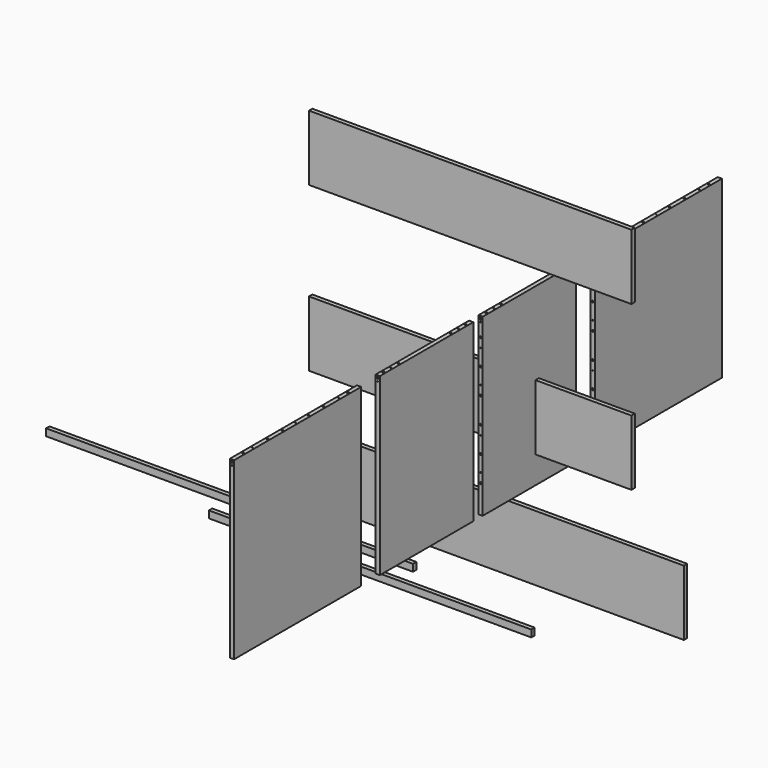
from build123d import *

# Parameters (mm, degrees)
F0_W      = 500
F0_H      = 750
F3_DEPTH  = 18
F4_D      = 4.5
F4_DEPTH  = 10
F4_TIP    = 1.3519363928
F5_D      = 8
F5_DEPTH  = 10
F5_TIP    = 2.4034424761
F6_D      = 5
F6_DEPTH  = 10
F6_TIP    = 1.5021515476
F7_W      = 680
F7_H      = 750
F8_DEPTH  = 18
F10_D     = 4
F11_D     = 8
F12_W     = 1570
F12_H     = 280
F13_DEPTH = 18
F14_W     = 1570
F14_H     = 280
F15_DEPTH = 18
F14_W_2   = 1380
F18_D     = 8
F18_DEPTH = 20
F18_TIP   = 2.4034424761
F19_D     = 5
F19_DEPTH = 60
F19_TIP   = 1.5021515476
F21_D     = 4
F21_DEPTH = 40
F21_TIP   = 1.2017212381
F22_D     = 8
F22_DEPTH = 30
F22_TIP   = 2.4034424761
F24_W     = 1570
F24_H     = 30
F25_DEPTH = 18
F27_D     = 8
F27_DEPTH = 10
F27_TIP   = 2.4034424761
F28_D     = 4
F28_DEPTH = 10
F28_TIP   = 1.2017212381
F29_W     = 1380
F29_H     = 30
F30_DEPTH = 18
F32_D     = 4
F32_DEPTH = 10
F32_TIP   = 1.2017212381
F33_D     = 8
F33_DEPTH = 10
F33_TIP   = 2.4034424761
F35_D     = 8
F35_DEPTH = 20
F35_TIP   = 2.4034424761
F36_D     = 4
F36_DEPTH = 40
F36_TIP   = 1.2017212381
F38_D     = 8
F39_D     = 4
F41_D     = 4
F41_DEPTH = 40
F41_START = 600
F41_TIP   = 1.2017212381
F42_D     = 8
F42_DEPTH = 25
F42_START = 600
F42_TIP   = 2.4034424761
F45_D     = 8
F45_DEPTH = 10
F45_TIP   = 2.4034424761
F46_D     = 8
F46_DEPTH = 10
F46_TIP   = 2.4034424761
F47_D     = 4
F47_DEPTH = 12
F47_TIP   = 1.2017212381
F48_D     = 4
F48_DEPTH = 12
F48_TIP   = 1.2017212381


# Not quite as in the source:
# - a feature names something its author has since deleted; it is built from what else it names


with BuildPart() as f3:
    # F0 (on Right) → F3 (new body)
    with BuildSketch(Plane.YZ):
        with Locations((-50.6659869477, 62.4944338164)):
            Rectangle(F0_W, F0_H)
    extrude(amount=F3_DEPTH)

    # F4
    with Locations(Plane(origin=(0, 0, 0), x_dir=(0, 1, 0), z_dir=(-1, 0, 0))):
        with Locations((114.6340130523, 182.5055661836), (50.6340130523, 182.5055661836), (-162.4159869477, 182.5055661836), (-226.4159869477, 182.5055661836), (114.6340130523, 12.5055661836), (50.6340130523, 12.5055661836), (-162.4159869477, 12.5055661836), (-226.4159869477, 12.5055661836), (-226.4159869477, -157.4944338164), (-162.4159869477, -157.4944338164), (114.6340130523, -157.4944338164), (50.6340130523, -157.4944338164)):
            Hole(F4_D / 2, depth=F4_DEPTH)
            with Locations((0, 0, -(F4_DEPTH + F4_TIP / 2))):  # 118° drill point
                Cone(0, F4_D / 2, F4_TIP, mode=Mode.SUBTRACT)

    # F5
    with Locations(Plane(origin=(0, 0, 0), x_dir=(0, 1, 0), z_dir=(-1, 0, 0))):
        with Locations((-250.6659869477, 257.5055661836), (-150.6659869477, 257.5055661836), (-50.6659869477, 257.5055661836), (49.3340130523, 257.5055661836), (149.3340130523, 257.5055661836), (149.3340130523, -232.4944338164), (49.3340130523, -232.4944338164), (-50.6659869477, -232.4944338164), (-250.6659869477, -232.4944338164), (-150.6659869477, -232.4944338164)):
            Hole(F5_D / 2, depth=F5_DEPTH)
            with Locations((0, 0, -(F5_DEPTH + F5_TIP / 2))):  # 118° drill point
                Cone(0, F5_D / 2, F5_TIP, mode=Mode.SUBTRACT)

    # F6
    with Locations(Plane(origin=(0, 0, 0), x_dir=(0, 1, 0), z_dir=(-1, 0, 0))):
        with Locations((99.3340130523, 257.5055661836), (-200.6659869477, 257.5055661836), (99.3340130523, -232.4944338164), (-200.6659869477, -232.4944338164)):
            Hole(F6_D / 2, depth=F6_DEPTH)
            with Locations((0, 0, -(F6_DEPTH + F6_TIP / 2))):  # 118° drill point
                Cone(0, F6_D / 2, F6_TIP, mode=Mode.SUBTRACT)

    # F18
    with Locations(Plane.XY.offset(437.4944338164)):
        with Locations((9, 169.3340130523), (9, 89.3340130523), (9, -190.6659869477), (9, -270.6659869477)):
            Hole(F18_D / 2, depth=F18_DEPTH)
            with Locations((0, 0, -(F18_DEPTH + F18_TIP / 2))):  # 118° drill point
                Cone(0, F18_D / 2, F18_TIP, mode=Mode.SUBTRACT)

    # F19
    with Locations(Plane.XY.offset(437.4944338164)):
        with Locations((9, 129.3340130523), (9, -230.6659869477)):
            Hole(F19_D / 2, depth=F19_DEPTH)
            with Locations((0, 0, -(F19_DEPTH + F19_TIP / 2))):  # 118° drill point
                Cone(0, F19_D / 2, F19_TIP, mode=Mode.SUBTRACT)

    # F35
    with Locations(Plane.XZ.offset(300.6659869477)):
        with Locations((9, 357.4944338164), (9, 247.4944338164), (9, 137.4944338164), (9, -192.5055661836), (9, -82.5055661836), (9, 27.4944338164)):
            Hole(F35_D / 2, depth=F35_DEPTH)
            with Locations((0, 0, -(F35_DEPTH + F35_TIP / 2))):  # 118° drill point
                Cone(0, F35_D / 2, F35_TIP, mode=Mode.SUBTRACT)

    # F36
    with Locations(Plane.XZ.offset(300.6659869477)):
        with Locations((9, 317.4944338164), (9, 177.4944338164), (9, -12.5055661836), (9, -152.5055661836)):
            Hole(F36_D / 2, depth=F36_DEPTH)
            with Locations((0, 0, -(F36_DEPTH + F36_TIP / 2))):  # 118° drill point
                Cone(0, F36_D / 2, F36_TIP, mode=Mode.SUBTRACT)

    # F38 (through all)
    with Locations(Plane(origin=(0, 199.3340130523, 0), x_dir=(-1, 0, 0), z_dir=(0, 1, 0))):
        with Locations((-9, 428.4944338164)):
            Hole(F38_D / 2)

    # F39 (through all)
    with Locations(Plane(origin=(0, 199.3340130523, 0), x_dir=(-1, 0, 0), z_dir=(0, 1, 0))):
        with Locations((-9, 414.9944338164)):
            Hole(F39_D / 2)


with BuildPart() as f8:
    # F7 (on Right) → F8 (new body)
    with BuildSketch(Plane.YZ):
        with Locations((639.3340130523, 62.4944338164)):
            Rectangle(F7_W, F7_H)
    extrude(amount=F8_DEPTH)

    # F10 (through all)
    with Locations(Plane(origin=(0, 979.3340130523, 0), x_dir=(-1, 0, 0), z_dir=(0, 1, 0))):
        with Locations((-9, 414.9944338164)):
            Hole(F10_D / 2)

    # F11 (through all)
    with Locations(Plane(origin=(0, 979.3340130523, 0), x_dir=(-1, 0, 0), z_dir=(0, 1, 0))):
        with Locations((-9, 428.4944338164)):
            Hole(F11_D / 2)

    # F21
    with Locations(Plane.XY.offset(437.4944338164)):
        with Locations((9, 869.3340130523), (9, 639.3340130523), (9, 409.3340130523)):
            Hole(F21_D / 2, depth=F21_DEPTH)
            with Locations((0, 0, -(F21_DEPTH + F21_TIP / 2))):  # 118° drill point
                Cone(0, F21_D / 2, F21_TIP, mode=Mode.SUBTRACT)

    # F22
    with Locations(Plane.XY.offset(437.4944338164)):
        with Locations((9, 359.3340130523), (9, 489.3340130523), (9, 569.3340130523), (9, 709.3340130523), (9, 789.3340130523), (9, 919.3340130523)):
            Hole(F22_D / 2, depth=F22_DEPTH)
            with Locations((0, 0, -(F22_DEPTH + F22_TIP / 2))):  # 118° drill point
                Cone(0, F22_D / 2, F22_TIP, mode=Mode.SUBTRACT)

    # F41
    # its depths count from where the whole tool has entered the part; down to there all is cleared
    with Locations(Plane.XZ.offset(300.6659869477)):
        with Locations((9, 317.4944338164), (9, 177.4944338164), (9, -12.5055661836), (9, -152.5055661836)):
            Hole(F41_D / 2, depth=F41_START)
    with Locations(Plane.XZ.offset(300.6659869477).offset(-F41_START)):
        with Locations((9, 317.4944338164), (9, 177.4944338164), (9, -12.5055661836), (9, -152.5055661836)):
            Hole(F41_D / 2, depth=F41_DEPTH)
            with Locations((0, 0, -(F41_DEPTH + F41_TIP / 2))):  # 118° drill point
                Cone(0, F41_D / 2, F41_TIP, mode=Mode.SUBTRACT)

    # F42
    # its depths count from where the whole tool has entered the part; down to there all is cleared
    with Locations(Plane.XZ.offset(300.6659869477)):
        with Locations((9, 357.4944338164), (9, 247.4944338164), (9, 137.4944338164), (9, 27.4944338164), (9, -82.5055661836), (9, -192.5055661836)):
            Hole(F42_D / 2, depth=F42_START)
    with Locations(Plane.XZ.offset(300.6659869477).offset(-F42_START)):
        with Locations((9, 357.4944338164), (9, 247.4944338164), (9, 137.4944338164), (9, 27.4944338164), (9, -82.5055661836), (9, -192.5055661836)):
            Hole(F42_D / 2, depth=F42_DEPTH)
            with Locations((0, 0, -(F42_DEPTH + F42_TIP / 2))):  # 118° drill point
                Cone(0, F42_D / 2, F42_TIP, mode=Mode.SUBTRACT)


with BuildPart() as f13:
    # F12 (on Front) → F13 (new body)
    with BuildSketch(Plane.XZ):
        with Locations((-131.9031941891, -548.7108457167)):
            Rectangle(F12_W, F12_H)
    extrude(amount=F13_DEPTH)

    # F46
    with Locations(Plane(origin=(0, 0, 0), x_dir=(-1, 0, 0), z_dir=(0, 1, 0))):
        with Locations((-644.0968058109, -438.7108457167), (-644.0968058109, -548.7108457167), (-644.0968058109, -658.7108457167), (907.9031941891, -438.7108457167), (907.9031941891, -548.7108457167), (907.9031941891, -658.7108457167)):
            Hole(F46_D / 2, depth=F46_DEPTH)
            with Locations((0, 0, -(F46_DEPTH + F46_TIP / 2))):  # 118° drill point
                Cone(0, F46_D / 2, F46_TIP, mode=Mode.SUBTRACT)

    # F47
    with Locations(Plane(origin=(0, 0, 0), x_dir=(-1, 0, 0), z_dir=(0, 1, 0))):
        with Locations((-644.0968058109, -478.7108457167), (-644.0968058109, -618.7108457167), (907.9031941891, -618.7108457167), (907.9031941891, -478.7108457167)):
            Hole(F47_D / 2, depth=F47_DEPTH)
            with Locations((0, 0, -(F47_DEPTH + F47_TIP / 2))):  # 118° drill point
                Cone(0, F47_D / 2, F47_TIP, mode=Mode.SUBTRACT)


with BuildPart() as f15:
    # F14 (on Front) → F15 (new body)
    with BuildSketch(Plane.XZ):
        with Locations((-131.9031941891, -548.7108457167)):
            Rectangle(F14_W, F14_H)
    extrude(amount=F15_DEPTH)


with BuildPart() as f15b:
    # F14 (on Front) → F15, piece 2 (new body)
    with BuildSketch(Plane.XZ):
        with Locations((-261.5306949615, -56.0900127888)):
            Rectangle(F14_W_2, F14_H)
    extrude(amount=F15_DEPTH)

    # F45
    with Locations(Plane(origin=(0, 0, 0), x_dir=(-1, 0, 0), z_dir=(0, 1, 0))):
        with Locations((-419.4693050385, 53.9099872112), (-419.4693050385, -56.0900127888), (-419.4693050385, -166.0900127888), (942.5306949615, -166.0900127888), (942.5306949615, -56.0900127888), (942.5306949615, 53.9099872112)):
            Hole(F45_D / 2, depth=F45_DEPTH)
            with Locations((0, 0, -(F45_DEPTH + F45_TIP / 2))):  # 118° drill point
                Cone(0, F45_D / 2, F45_TIP, mode=Mode.SUBTRACT)

    # F48
    with Locations(Plane(origin=(0, 0, 0), x_dir=(-1, 0, 0), z_dir=(0, 1, 0))):
        with Locations((-419.4693050385, 13.9099872112), (-419.4693050385, -126.0900127888), (942.5306949615, -126.0900127888), (942.5306949615, 13.9099872112)):
            Hole(F48_D / 2, depth=F48_DEPTH)
            with Locations((0, 0, -(F48_DEPTH + F48_TIP / 2))):  # 118° drill point
                Cone(0, F48_D / 2, F48_TIP, mode=Mode.SUBTRACT)


with BuildPart() as f25:
    # F24 (on Front) → F25 (new body)
    with BuildSketch(Plane.XZ):
        with Locations((-1291.3920255528, -793.7992012501)):
            Rectangle(F24_W, F24_H)
    extrude(amount=F25_DEPTH)

    # F27
    with Locations(Plane(origin=(0, 0, 0), x_dir=(-1, 0, 0), z_dir=(0, 1, 0))):
        with Locations((2067.3920255528, -787.7992012501), (515.3920255528, -787.7992012501)):
            Hole(F27_D / 2, depth=F27_DEPTH)
            with Locations((0, 0, -(F27_DEPTH + F27_TIP / 2))):  # 118° drill point
                Cone(0, F27_D / 2, F27_TIP, mode=Mode.SUBTRACT)

    # F28
    with Locations(Plane(origin=(0, 0, 0), x_dir=(-1, 0, 0), z_dir=(0, 1, 0))):
        with Locations((515.3920255528, -801.2992012501), (2067.3920255528, -801.2992012501)):
            Hole(F28_D / 2, depth=F28_DEPTH)
            with Locations((0, 0, -(F28_DEPTH + F28_TIP / 2))):  # 118° drill point
                Cone(0, F28_D / 2, F28_TIP, mode=Mode.SUBTRACT)


with BuildPart() as f30:
    # F29 (on Front) → F30 (new body)
    with BuildSketch(Plane.XZ):
        with Locations((-690, -876.5716409683)):
            Rectangle(F29_W, F29_H)
    extrude(amount=F30_DEPTH)

    # F32
    with Locations(Plane(origin=(0, 0, 0), x_dir=(-1, 0, 0), z_dir=(0, 1, 0))):
        with Locations((9, -884.0716409683), (1371, -884.0716409683)):
            Hole(F32_D / 2, depth=F32_DEPTH)
            with Locations((0, 0, -(F32_DEPTH + F32_TIP / 2))):  # 118° drill point
                Cone(0, F32_D / 2, F32_TIP, mode=Mode.SUBTRACT)

    # F33
    with Locations(Plane(origin=(0, 0, 0), x_dir=(-1, 0, 0), z_dir=(0, 1, 0))):
        with Locations((9, -870.5716409683), (1371, -870.5716409683)):
            Hole(F33_D / 2, depth=F33_DEPTH)
            with Locations((0, 0, -(F33_DEPTH + F33_TIP / 2))):  # 118° drill point
                Cone(0, F33_D / 2, F33_TIP, mode=Mode.SUBTRACT)


with BuildPart() as f40_1:
    # F40: instance of F3
    add(f3.part.mirror(Plane(origin=(9, -325.6659869477, 62.4944338164), x_dir=(1, 0, 0), z_dir=(0, -1, 0))))


with BuildPart() as f43_1:
    # F43: instance of F8
    add(f8.part.mirror(Plane(origin=(9, -325.6659869477, 62.4944338164), x_dir=(1, 0, 0), z_dir=(0, -1, 0))))


with BuildPart() as f49_1:
    # F49: copy of F15b
    add(f15b.part.moved(Location((0, 0, 700))))


solid = Compound([f3.part, f8.part, f13.part, f15b.part, f25.part, f30.part, f40_1.part, f43_1.part, f49_1.part])
